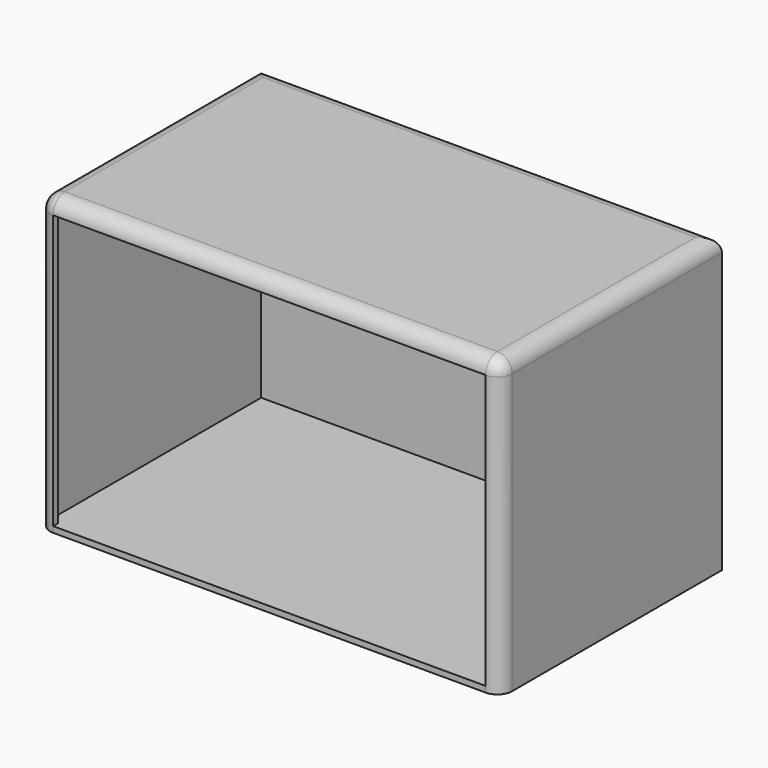
from build123d import *

# Parameters (mm, degrees)
F0_W     = 199.3581205606
F0_H     = 119.528003037
F1_DEPTH = 127
F2_R     = 6.35
F3_T     = -2.54


# Not quite as in the source:
# - a shell that OpenCascade refuses in one call is made with other operations: the cavity is built on its own and cut out


with BuildPart() as f1:
    # F0 (on Top) → F1 (new body)
    with BuildSketch(Plane.XY):
        with Locations((-20.9509953856, 1.4819204807)):
            Rectangle(F0_W, F0_H)
    extrude(amount=F1_DEPTH)

    # F2
    f2_edges = [f1.edges().sort_by_distance(p)[0] for p in [
        (-20.950995, -58.282081, 127),
        (78.728065, 1.48192, 127),
        (-20.950995, 61.245922, 127),
        (-120.630056, 1.48192, 127),
        (-120.630056, -58.282081, 63.5),
        (78.728065, -58.282081, 63.5),
    ]]
    fillet(f2_edges, radius=F2_R)

    # F3: a shell. OpenCascade refuses it in one call, so the cavity is built on its own and cut out:
    # the body offset inwards by the wall thickness, plus a prism from it out through each open face.
    f3_core = offset(f1.part, amount=F3_T, mode=Mode.PRIVATE)
    f3_exits = [f3_core.faces().sort_by_distance(p)[0] for p in [
        (-20.950995, -55.742081, 61.595),
    ]]
    add(f3_core, mode=Mode.SUBTRACT)
    extrude(f3_exits, amount=-F3_T, mode=Mode.SUBTRACT)


solid = f1.part
